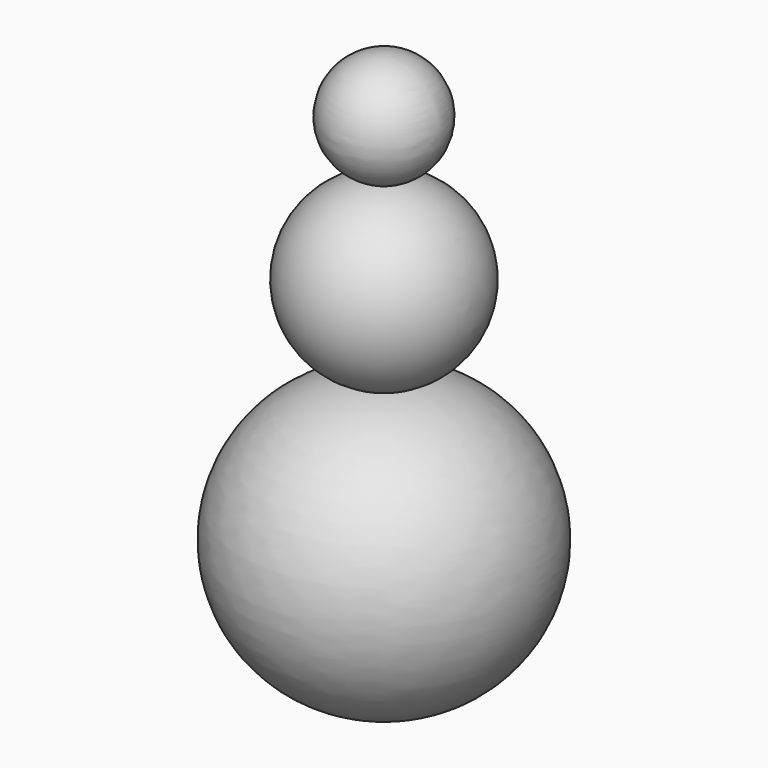
from build123d import *

# Parameters (mm, degrees)
F2_R     = 1.0641522899
F2_R_2   = 1.2861157266
F3_DEPTH = 25.4


with BuildPart() as f1:
    # F0 (on Front) → F1 (revolve)
    with BuildSketch(Plane.XZ):
        with BuildLine():
            ThreePointArc((0.4812036321, 0.0113761322), (0.2406690424, 0.0028444303), (0, 0))
            Line((0, 0), (0, -32.0318564773))
            ThreePointArc((0, -32.0318564773), (16.6454616461, -16.256597281), (0.4812036321, 0.0113761322))
        make_face()
    revolve(axis=Axis((0, 0, -16.0159282386), (0, 0, -1)))


with BuildPart() as f1b:
    # F0 (on Front) → F1, piece 2 (revolve)
    with BuildSketch(Plane.XZ):
        with BuildLine():
            Line((0, 20.3660037369), (0, 0))
            ThreePointArc((0, 0), (0.2405591087, 0.0074945621), (0.4812036321, 0.0113761322))
            ThreePointArc((0.4812036321, 0.0113761322), (10.1810110476, 10.3843500772), (0.0786594626, 20.3656999265))
            ThreePointArc((0.0786594626, 20.3656999265), (0.039329253, 20.3657279925), (0, 20.3660037369))
        make_face()
        with BuildLine():
            ThreePointArc((0.0786594626, 20.3656999265), (0.0393300247, 20.365927784), (0, 20.3660037369))
            ThreePointArc((0, 20.3660037369), (0.039329253, 20.3657279925), (0.0786594626, 20.3656999265))
        make_face()
        with BuildLine():
            Line((0, 32.8561924398), (0, 20.3660037369))
            ThreePointArc((0, 20.3660037369), (0.0393300247, 20.365927784), (0.0786594626, 20.3656999265))
            ThreePointArc((0.0786594626, 20.3656999265), (6.3087438977, 26.650428113), (0, 32.8561924398))
        make_face()
    revolve(axis=Axis((0, 0, -16.0159282386), (0, 0, -1)))

    # F2 (on Front) → F3 (cut)
    with BuildSketch(Plane.XZ):
        with Locations((-2.8087825049, 28.8563799113)):
            Circle(F2_R)
        with Locations((2.7184134815, 28.8563799113)):
            Circle(F2_R_2)
        with BuildLine():
            Line((3.2824131195, 24.682784453), (-3.5983817652, 24.682784453))
            ThreePointArc((-3.5983817652, 24.682784453), (-0.1579843229, 22.5582328984), (3.2824131195, 24.682784453))
        make_face()
    extrude(amount=-F3_DEPTH, mode=Mode.SUBTRACT)


solid = Compound([f1.part, f1b.part])
